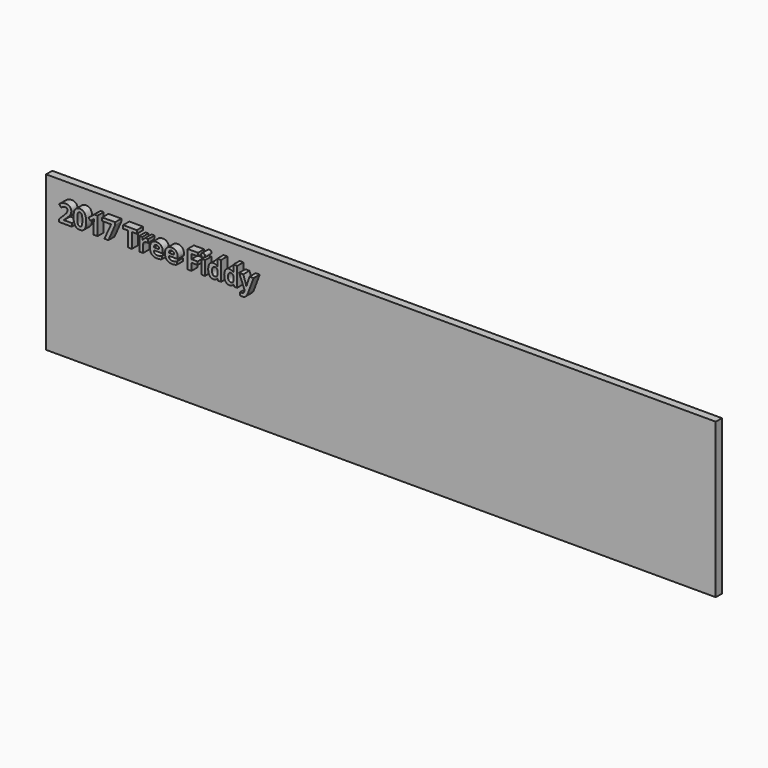
from build123d import *

# Parameters (mm, degrees)
F0_W         = 65
F0_H         = 30
F1_DEPTH     = 1.5
F2_TEXT_SIZE = 4.9237537548
F3_DEPTH     = 1.5


# Not quite as in the source:
# - Text() gives the source's letters only with a copy of the font that has no kerning and outlines rounded to 1/6400 em; it was checked with that copy


with BuildPart() as f1:
    # F0 (on Front) → F1 (new body)
    with BuildSketch(Plane.XZ):
        with Locations((32.5, 15)):
            Rectangle(F0_W, F0_H)
        with Locations((-32.5, 15)):
            Rectangle(F0_W, F0_H)
    extrude(amount=F1_DEPTH)

    # F2 (on face) → F3 (join)
    with BuildSketch(Plane.XZ.offset(1.5)):
        with Locations((-61.4609960732, 23.6730083508)):
            Text('2017 Tree Fiddy', F2_TEXT_SIZE, font='Open Sans', font_style=FontStyle.BOLD, text_align=(TextAlign.LEFT, TextAlign.BOTTOM))
    extrude(amount=F3_DEPTH)


solid = f1.part
